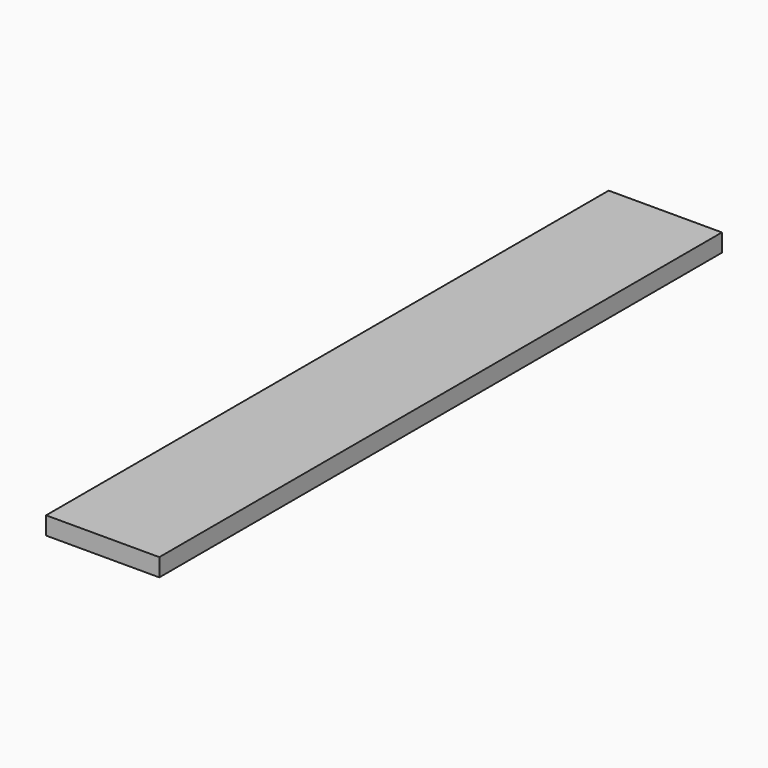
from build123d import *

# Parameters (mm, degrees)
F0_W     = 80.518
F0_H     = 499.999
F1_DEPTH = 6.35
F2_W     = 67.818
F2_H     = 6.35
F3_DEPTH = 6.35
F5_DEPTH = 6.35
F6_DEPTH = 6.35
F7_DEPTH = 6.35


# Not quite as in the source:
# - a feature names something its author has since deleted; it is built from what else it names


with BuildPart() as f1:
    # F0 (on Top) → F1 (new body)
    with BuildSketch(Plane.XY):
        with Locations((40.259, 230.6542872722)):
            Rectangle(F0_W, F0_H)
    extrude(amount=F1_DEPTH)

    # F2 (on face) → F3 (join)
    with BuildSketch(Plane(origin=(0, 0, 0), x_dir=(1, 0, 0), z_dir=(0, 0, -1))):
        Polygon((80.518, 19.3452127278), (74.168, 19.3452127278), (74.168, 12.9952127278), (74.168, -474.3037872722), (74.168, -480.6537872722), (80.518, -480.6537872722), align=None)
        Polygon((6.35, 19.3452127278), (0, 19.3452127278), (0, -480.6537872722), (6.35, -480.6537872722), (6.35, -474.3037872722), (6.35, 12.9952127278), align=None)
        with Locations((40.259, 16.1702127278)):
            Rectangle(F2_W, F2_H)
        with Locations((40.259, -477.4787872722)):
            Rectangle(F2_W, F2_H)
    extrude(amount=F3_DEPTH)

    # F4 (on face) → F5 (join)
    with BuildSketch(Plane(origin=(0, 0, 0), x_dir=(1, 0, 0), z_dir=(0, 0, -1))):
        Polygon((43.434, 12.9952127278), (37.084, 12.9952127278), (37.084, -7.4495371679), (37.084, -27.9419109224), (37.084, -69.0037844682), (37.084, -89.3237844682), (37.084, -130.4718448913), (37.084, -150.7918448913), (37.084, -191.9399053144), (37.084, -212.2599053144), (37.084, -253.4079657375), (37.084, -263.5679657375), (37.084, -273.7279657375), (37.084, -314.8760261606), (37.084, -335.1960261606), (37.084, -376.3440865837), (37.084, -386.5040865837), (37.084, -396.6640865837), (37.084, -437.8136164283), (37.084, -458.1321470068), (37.084, -474.3037872722), (43.434, -474.3037872722), (43.434, -457.6869668698), (43.434, -437.3826820421), (43.434, -396.2331521975), (43.434, -386.0731521975), (43.434, -375.9131521975), (43.434, -334.8512786517), (43.434, -314.3589048972), (43.434, -273.4694051058), (43.434, -263.2232182286), (43.434, -252.9770313513), (43.434, -212.08753156), (43.434, -191.5951578055), (43.434, -150.6912914171), (43.434, -130.2132842596), (43.434, -89.3237844682), (43.434, -68.8314107138), (43.434, -27.9419109224), (43.434, -7.5214582917), align=None)
        Polygon((48.5570884026, -319.4891816343), (43.434, -314.3589048972), (43.434, -334.8512786517), (48.5570884026, -329.7210019146), (74.168, -355.2960285474), (74.168, -345.1360285474), (53.6658303382, -324.6050917744), (74.168, -304.0741550015), (74.168, -293.9141550015), align=None)
        Polygon((48.5132602963, -442.4548254861), (43.434, -437.3826820421), (43.434, -457.6869668698), (48.5139950064, -452.6140897452), (70.2341258947, -474.3037872722), (74.168, -474.3037872722), (74.168, -468.0736188151), (53.5932553027, -447.5277026107), (74.168, -426.9240889705), (74.168, -416.7640889705), align=None)
        Polygon((37.084, -458.1321470068), (37.084, -437.8136164283), (32.0047397037, -442.8857598723), (6.35, -417.1950233567), (6.35, -427.3550233567), (26.9247446973, -447.9586369969), (6.35, -468.5045532013), (6.35, -474.3037872722), (10.7154131464, -474.3037872722), (32.0040049936, -453.0450241314), align=None)
        Polygon((6.35, -417.1950233567), (32.0040049936, -391.5769637083), (26.9240099873, -386.4898408329), (6.35, -407.0350233567), align=None)
        Polygon((53.5939900127, -386.0589064467), (48.5139950064, -391.1460293221), (74.168, -416.7640889705), (74.168, -406.6040889705), align=None)
        Polygon((48.5570884026, -196.7254345426), (43.434, -191.5951578055), (43.434, -212.08753156), (48.5570884026, -206.9572548229), (74.168, -232.5322814557), (74.168, -222.3722814557), (53.6658303382, -201.8413446827), (74.168, -181.3104079098), (74.168, -171.1504079098), align=None)
        Polygon((74.168, -232.5322814557), (48.5570884026, -258.1073080885), (53.6658303382, -263.2232182286), (74.168, -242.6922814557), align=None)
        Polygon((37.084, -335.1960261606), (37.084, -314.8760261606), (32.0040049936, -319.9489032852), (6.35, -294.2589025105), (6.35, -304.4189025105), (26.9240099873, -325.0217804098), (6.35, -345.5669629336), (6.35, -355.7269629336), (32.0040049936, -330.1089032852), align=None)
        Polygon((26.9240099873, -263.5537199867), (32.0040049936, -258.4808428621), (6.35, -232.7908420874), (6.35, -242.9508420874), align=None)
    extrude(amount=F5_DEPTH)

    # F4 (on face) → F6 (join)
    with BuildSketch(Plane(origin=(0, 0, 0), x_dir=(1, 0, 0), z_dir=(0, 0, -1))):
        Polygon((37.084, -150.7918448913), (37.084, -130.4718448913), (32.0040049936, -135.5447220159), (6.35, -109.8547212412), (6.35, -120.0147212412), (26.9240099873, -140.6175991405), (6.35, -161.1627816643), (6.35, -171.3227816643), (32.0040049936, -145.7047220159), align=None)
        Polygon((48.5570884026, -135.3435609967), (43.434, -130.2132842596), (43.434, -150.6912914171), (48.5570884026, -145.575381277), (74.168, -171.1504079098), (74.168, -160.9904079098), (53.6658303382, -140.4594711369), (74.168, -119.9285343639), (74.168, -109.7685343639), align=None)
        Polygon((31.9609115974, -12.579813905), (6.35, 12.9952127278), (6.35, 2.8352127278), (26.8521696618, -17.6957240451), (6.35, -38.2266608181), (6.35, -48.3866608181), (31.9609115974, -22.8116341853), (37.084, -27.9419109224), (37.084, -7.4495371679), align=None)
        Polygon((74.168, 2.8352127278), (74.168, 12.9952127278), (48.5211278761, -12.6157240451), (43.434, -7.5214582917), (43.434, -27.9419109224), (48.5570884026, -22.8116341853), (74.168, -48.3866608181), (74.168, -38.2266608181), (53.637083409, -17.7245113099), align=None)
        Polygon((48.5570884026, -73.9616874509), (43.434, -68.8314107138), (43.434, -89.3237844682), (48.5570884026, -84.1935077311), (74.168, -109.7685343639), (74.168, -99.6085343639), (53.6658303382, -79.077597591), (74.168, -58.5466608181), (74.168, -48.3866608181), align=None)
    extrude(amount=F6_DEPTH)

    # F4 (on face) → F7 (join)
    with BuildSketch(Plane(origin=(0, 0, 0), x_dir=(1, 0, 0), z_dir=(0, 0, -1))):
        Polygon((32.0040049936, -74.0766615928), (6.35, -48.3866608181), (6.35, -58.5466608181), (26.9240099873, -79.1495387174), (6.35, -99.6947212412), (6.35, -109.8547212412), (32.0040049936, -84.2366615928), (37.084, -89.3237844682), (37.084, -69.0037844682), align=None)
        Polygon((37.084, -212.2599053144), (37.084, -191.9399053144), (32.0040049936, -197.012782439), (6.35, -171.3227816643), (6.35, -181.4827816643), (26.9240099873, -202.0856595636), (6.35, -222.6308420874), (6.35, -232.7908420874), (32.0040049936, -207.172782439), align=None)
    extrude(amount=F7_DEPTH)


solid = f1.part
